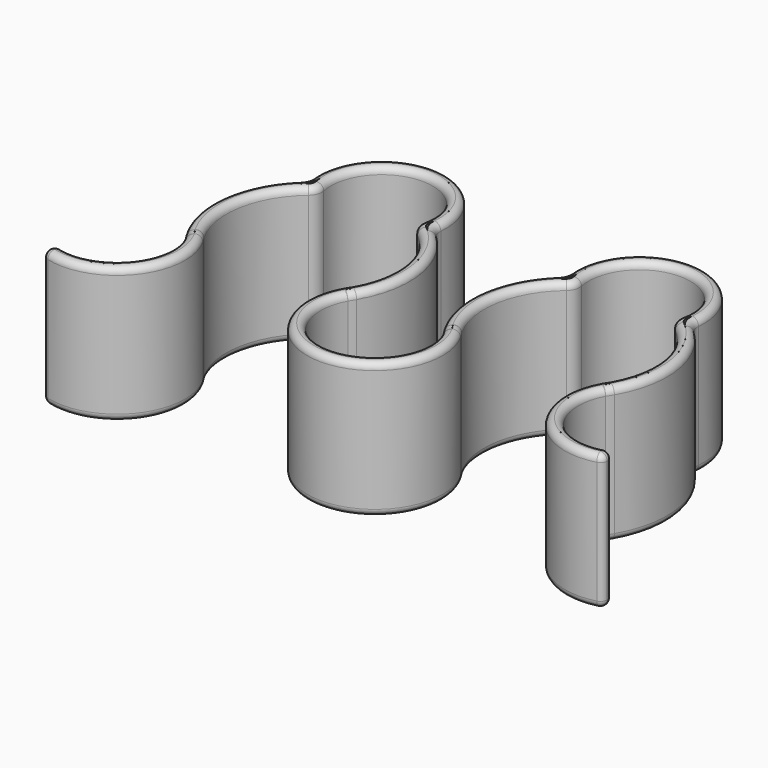
from build123d import *

# Parameters (mm, degrees)
F1_DEPTH = 20
F2_R     = 0.9999
F3_R     = 0.9999


# Not quite as in the source:
# - a fillet or chamfer is up to 0.001 mm smaller than in the source, because OpenCascade refuses the exact size


with BuildPart() as f1:
    # F0 (on Top) → F1 (new body)
    with BuildSketch(Plane.XY):
        with BuildLine():
            ThreePointArc((-7.0345135957, 3.8099368068), (-6.7639112242, 4.2719439311), (-6.4630111568, 4.7148156685))
            ThreePointArc((-6.4630111568, 4.7148156685), (-4.6396535759, 14.0075982117), (-8.9415858388, 22.4440559441))
            ThreePointArc((-8.9415858388, 22.4440559441), (-9.4305302676, 23.1921894632), (-9.5447890869, 24.0785953177))
            ThreePointArc((-9.5447890869, 24.0785953177), (-19, 34.5), (-28.4552109131, 24.0785953177))
            ThreePointArc((-28.4552109131, 24.0785953177), (-28.5694697324, 23.1921894632), (-29.0584141612, 22.4440559441))
            ThreePointArc((-29.0584141612, 22.4440559441), (-33.3603464241, 14.0075982117), (-31.5369888432, 4.7148156685))
            ThreePointArc((-31.5369888432, 4.7148156685), (-31.2360887758, 4.2719439311), (-30.9654864043, 3.8099368068))
            ThreePointArc((-30.9654864043, 3.8099368068), (-31.6885763695, -4.9158856533), (-39.9718481965, -7.7531809401))
            ThreePointArc((-39.9718481965, -7.7531809401), (-40.8321365912, -7.9328727246), (-41.218329221, -8.7223285576))
            ThreePointArc((-41.218329221, -8.7223285576), (-41.007785054, -9.3361359278), (-40.4648102456, -9.6914761751))
            ThreePointArc((-40.4648102456, -9.6914761751), (-30.0759546476, -6.0999594469), (-29.2615101333, 4.8619743778))
            ThreePointArc((-29.2615101333, 4.8619743778), (-29.5686112879, 5.3250876077), (-29.8548265003, 5.8013919589))
            ThreePointArc((-29.8548265003, 5.8013919589), (-31.3040020891, 14.2048883398), (-27.0268863403, 21.5822281167))
            ThreePointArc((-27.0268863403, 21.5822281167), (-26.4236170012, 22.4542680293), (-26.3509380169, 23.512145749))
            ThreePointArc((-26.3509380169, 23.512145749), (-19, 32.5), (-11.6490619831, 23.512145749))
            ThreePointArc((-11.6490619831, 23.512145749), (-11.5763829988, 22.4542680293), (-10.9731136597, 21.5822281167))
            ThreePointArc((-10.9731136597, 21.5822281167), (-6.6959979109, 14.2048883398), (-8.1451734997, 5.8013919589))
            ThreePointArc((-8.1451734997, 5.8013919589), (-8.4313887121, 5.3250876077), (-8.7384898667, 4.8619743778))
            ThreePointArc((-8.7384898667, 4.8619743778), (0, -10), (8.7384898667, 4.8619743778))
            ThreePointArc((8.7384898667, 4.8619743778), (8.4313887121, 5.3250876077), (8.1451734997, 5.8013919589))
            ThreePointArc((8.1451734997, 5.8013919589), (6.6959979109, 14.2048883398), (10.9731136597, 21.5822281167))
            ThreePointArc((10.9731136597, 21.5822281167), (11.5763829988, 22.4542680293), (11.6490619831, 23.512145749))
            ThreePointArc((11.6490619831, 23.512145749), (19, 32.5), (26.3509380169, 23.512145749))
            ThreePointArc((26.3509380169, 23.512145749), (26.4236170012, 22.4542680293), (27.0268863403, 21.5822281167))
            ThreePointArc((27.0268863403, 21.5822281167), (31.3040020891, 14.2048883398), (29.8548265003, 5.8013919589))
            ThreePointArc((29.8548265003, 5.8013919589), (29.5686112879, 5.3250876077), (29.2615101333, 4.8619743778))
            ThreePointArc((29.2615101333, 4.8619743778), (30.0759546476, -6.0999594469), (40.4648102456, -9.6914761751))
            ThreePointArc((40.4648102456, -9.6914761751), (41.007785054, -9.3361359278), (41.218329221, -8.7223285576))
            ThreePointArc((41.218329221, -8.7223285576), (40.8321365912, -7.9328727246), (39.9718481965, -7.7531809401))
            ThreePointArc((39.9718481965, -7.7531809401), (31.6885763695, -4.9158856533), (30.9654864043, 3.8099368068))
            ThreePointArc((30.9654864043, 3.8099368068), (31.2360887758, 4.2719439311), (31.5369888432, 4.7148156685))
            ThreePointArc((31.5369888432, 4.7148156685), (33.3603464241, 14.0075982117), (29.0584141612, 22.4440559441))
            ThreePointArc((29.0584141612, 22.4440559441), (28.5694697324, 23.1921894632), (28.4552109131, 24.0785953177))
            ThreePointArc((28.4552109131, 24.0785953177), (19, 34.5), (9.5447890869, 24.0785953177))
            ThreePointArc((9.5447890869, 24.0785953177), (9.4305302676, 23.1921894632), (8.9415858388, 22.4440559441))
            ThreePointArc((8.9415858388, 22.4440559441), (4.6396535759, 14.0075982117), (6.4630111568, 4.7148156685))
            ThreePointArc((6.4630111568, 4.7148156685), (6.7639112242, 4.2719439311), (7.0345135957, 3.8099368068))
            ThreePointArc((7.0345135957, 3.8099368068), (0, -8), (-7.0345135957, 3.8099368068))
        make_face()
        with BuildLine():
            ThreePointArc((-30.9654864043, 3.8099368068), (-31.2360887758, 4.2719439311), (-31.5369888432, 4.7148156685))
            ThreePointArc((-31.5369888432, 4.7148156685), (-31.2595890939, 4.2571016249), (-30.9654864043, 3.8099368068))
        make_face()
        with BuildLine():
            ThreePointArc((6.4630111568, 4.7148156685), (6.7404109061, 4.2571016249), (7.0345135957, 3.8099368068))
            ThreePointArc((7.0345135957, 3.8099368068), (6.7639112242, 4.2719439311), (6.4630111568, 4.7148156685))
        make_face()
        with BuildLine():
            ThreePointArc((-7.0345135957, 3.8099368068), (-6.7404109061, 4.2571016249), (-6.4630111568, 4.7148156685))
            ThreePointArc((-6.4630111568, 4.7148156685), (-6.7639112242, 4.2719439311), (-7.0345135957, 3.8099368068))
        make_face()
        with BuildLine():
            ThreePointArc((29.8548265003, 5.8013919589), (29.5451109697, 5.3399299139), (29.2615101333, 4.8619743778))
            ThreePointArc((29.2615101333, 4.8619743778), (29.5686112879, 5.3250876077), (29.8548265003, 5.8013919589))
        make_face()
        with BuildLine():
            ThreePointArc((30.9654864043, 3.8099368068), (31.2595890939, 4.2571016249), (31.5369888432, 4.7148156685))
            ThreePointArc((31.5369888432, 4.7148156685), (31.2360887758, 4.2719439311), (30.9654864043, 3.8099368068))
        make_face()
        with BuildLine():
            ThreePointArc((-8.7384898667, 4.8619743778), (-8.4313887121, 5.3250876077), (-8.1451734997, 5.8013919589))
            ThreePointArc((-8.1451734997, 5.8013919589), (-8.4548890303, 5.3399299139), (-8.7384898667, 4.8619743778))
        make_face()
        with BuildLine():
            ThreePointArc((8.1451734997, 5.8013919589), (8.4313887121, 5.3250876077), (8.7384898667, 4.8619743778))
            ThreePointArc((8.7384898667, 4.8619743778), (8.4548890303, 5.3399299139), (8.1451734997, 5.8013919589))
        make_face()
        with BuildLine():
            ThreePointArc((-29.8548265003, 5.8013919589), (-29.5686112879, 5.3250876077), (-29.2615101333, 4.8619743778))
            ThreePointArc((-29.2615101333, 4.8619743778), (-29.5451109697, 5.3399299139), (-29.8548265003, 5.8013919589))
        make_face()
    extrude(amount=F1_DEPTH)

    # F2 (radius 1 in the source; OpenCascade refuses exactly that, so slightly less here)
    f2_edges = [f1.edges().sort_by_distance(p)[0] for p in [
        (-29.749311, -5.650321, 20),
        (-31.304002, 14.204888, 20),
        (-26.423617, 22.454268, 20),
        (-19, 32.5, 20),
        (-11.576383, 22.454268, 20),
        (-6.695998, 14.204888, 20),
        (0, -10, 20),
        (6.695998, 14.204888, 20),
        (11.576383, 22.454268, 20),
        (19, 32.5, 20),
        (26.423617, 22.454268, 20),
        (31.304002, 14.204888, 20),
        (29.749311, -5.650321, 20),
        (41.187477, -8.475848, 20),
        (31.688576, -4.915886, 20),
        (33.424654, 13.476263, 20),
        (28.56947, 23.192189, 20),
        (19, 34.5, 20),
        (9.43053, 23.192189, 20),
        (4.575346, 13.476263, 20),
        (0, -8, 20),
        (-4.575346, 13.476263, 20),
        (-9.43053, 23.192189, 20),
        (-19, 34.5, 20),
        (-28.56947, 23.192189, 20),
        (-33.424654, 13.476263, 20),
        (-31.688576, -4.915886, 20),
        (-41.187477, -8.475848, 20),
    ]]
    fillet(f2_edges, radius=F2_R)

    # F3 (radius 1 in the source; OpenCascade refuses exactly that, so slightly less here)
    f3_edges = [f1.edges().sort_by_distance(p)[0] for p in [
        (-29.749311, -5.650321, 0),
        (-31.304002, 14.204888, 0),
        (-26.423617, 22.454268, 0),
        (-19, 32.5, 0),
        (-11.576383, 22.454268, 0),
        (-6.695998, 14.204888, 0),
        (0, -10, 0),
        (6.695998, 14.204888, 0),
        (11.576383, 22.454268, 0),
        (19, 32.5, 0),
        (26.423617, 22.454268, 0),
        (31.304002, 14.204888, 0),
        (29.749311, -5.650321, 0),
        (41.187477, -8.475848, 0),
        (31.688576, -4.915886, 0),
        (33.424654, 13.476263, 0),
        (28.56947, 23.192189, 0),
        (19, 34.5, 0),
        (9.43053, 23.192189, 0),
        (4.575346, 13.476263, 0),
        (0, -8, 0),
        (-4.575346, 13.476263, 0),
        (-9.43053, 23.192189, 0),
        (-19, 34.5, 0),
        (-28.56947, 23.192189, 0),
        (-33.424654, 13.476263, 0),
        (-31.688576, -4.915886, 0),
        (-41.187477, -8.475848, 0),
    ]]
    fillet(f3_edges, radius=F3_R)


solid = f1.part
